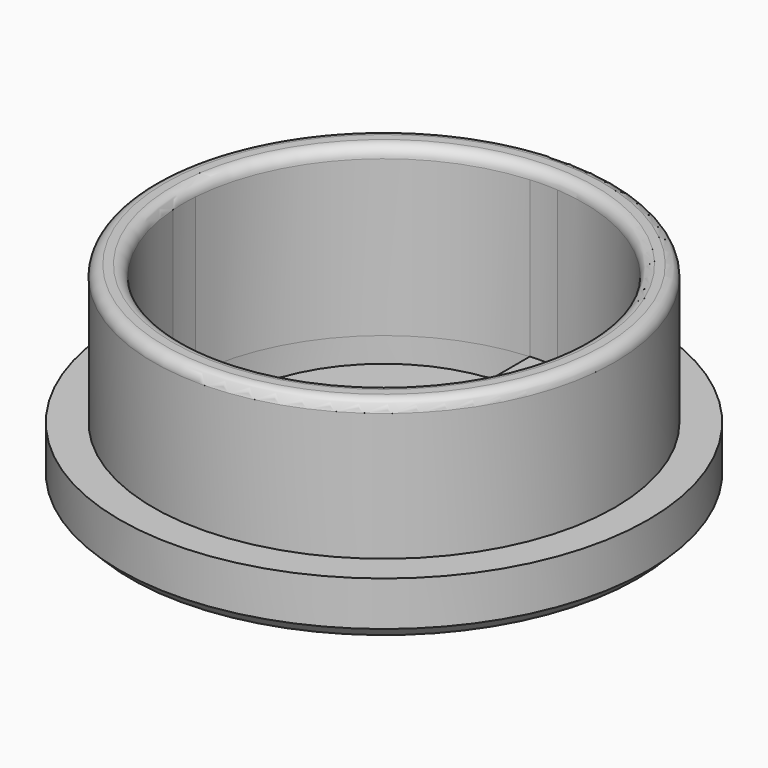
from build123d import *
from build123d import SkipClean  # not in build123d's __all__

# Parameters (mm, degrees)
F0_R     = 41.5
F0_R_2   = 36
F1_DEPTH = 35
F0_R_3   = 47.5
F2_DEPTH = 10
F3_DEPTH = 5
F4_R     = 2
F5_SIZE  = 2
F7_DEPTH = 40.1


with BuildPart() as f1:
    # F0 (on Top) → F1 (new body)
    with BuildSketch(Plane.XY):
        Circle(F0_R)
        Circle(F0_R_2, mode=Mode.SUBTRACT)
    extrude(amount=F1_DEPTH)

    # F0 (on Top) → F2 (join)
    with BuildSketch(Plane.XY):
        Circle(F0_R_3)
        Circle(F0_R, mode=Mode.SUBTRACT)
    extrude(amount=F2_DEPTH)

    # F0 (on Top) → F3 (join)
    with BuildSketch(Plane.XY):
        Circle(F0_R_2)
    extrude(amount=F3_DEPTH)

    # F4
    f4_edges = [f1.edges().sort_by_distance(p)[0] for p in [
        (-41.5, 0, 35),
        (-36, 0, 35),
    ]]
    fillet(f4_edges, radius=F4_R)

    # F5
    f5_edges = [f1.edges().sort_by_distance(p)[0] for p in [
        (-47.5, 0, 0),
    ]]
    chamfer(f5_edges, length=F5_SIZE)

    # F6 (on face) → F7 (cut)
    with BuildSketch(Plane.XY):
        with BuildLine():
            ThreePointArc((27.3098579389, -2.5), (19.3917294309, -19.3917294309), (2.5, -27.3098579389))
            Line((2.5, -27.3098579389), (2.5, -35.9130895357))
            ThreePointArc((2.5, -35.9130895357), (25.4558441227, -25.4558441227), (35.9130895357, -2.5))
            Line((35.9130895357, -2.5), (27.3098579389, -2.5))
        make_face()
        with BuildLine():
            Line((-2.5, -35.9130895357), (-2.5, -27.3098579389))
            ThreePointArc((-2.5, -27.3098579389), (-19.3917294309, -19.3917294309), (-27.3098579389, -2.5))
            Line((-27.3098579389, -2.5), (-35.9130895357, -2.5))
            ThreePointArc((-35.9130895357, -2.5), (-25.4558441227, -25.4558441227), (-2.5, -35.9130895357))
        make_face()
        with BuildLine():
            ThreePointArc((-27.3098579389, 2.5), (-19.3917294309, 19.3917294309), (-2.5, 27.3098579389))
            Line((-2.5, 27.3098579389), (-2.5, 35.9130895357))
            ThreePointArc((-2.5, 35.9130895357), (-25.4558441227, 25.4558441227), (-35.9130895357, 2.5))
            Line((-35.9130895357, 2.5), (-27.3098579389, 2.5))
        make_face()
        with BuildLine():
            Line((2.5, 35.9130895357), (2.5, 27.3098579389))
            ThreePointArc((2.5, 27.3098579389), (19.3917294309, 19.3917294309), (27.3098579389, 2.5))
            Line((27.3098579389, 2.5), (35.9130895357, 2.5))
            ThreePointArc((35.9130895357, 2.5), (25.4558441227, 25.4558441227), (2.5, 35.9130895357))
        make_face()
        with BuildLine():
            Line((2.5, 17.8404992818), (2.5, 8.7134999292))
            ThreePointArc((2.5, 8.7134999292), (6.4099563577, 6.4099563577), (8.7134999292, 2.5))
            Line((8.7134999292, 2.5), (17.8404992818, 2.5))
            ThreePointArc((17.8404992818, 2.5), (12.7383950053, 12.7383950053), (2.5, 17.8404992818))
        make_face()
        with BuildLine():
            ThreePointArc((8.7134999292, -2.5), (6.4099563577, -6.4099563577), (2.5, -8.7134999292))
            Line((2.5, -8.7134999292), (2.5, -17.8404992818))
            ThreePointArc((2.5, -17.8404992818), (12.7383950053, -12.7383950053), (17.8404992818, -2.5))
            Line((17.8404992818, -2.5), (8.7134999292, -2.5))
        make_face()
        with BuildLine():
            Line((-2.5, -17.8404992818), (-2.5, -8.7134999292))
            ThreePointArc((-2.5, -8.7134999292), (-6.4099563577, -6.4099563577), (-8.7134999292, -2.5))
            Line((-8.7134999292, -2.5), (-17.8404992818, -2.5))
            ThreePointArc((-17.8404992818, -2.5), (-12.7383950053, -12.7383950053), (-2.5, -17.8404992818))
        make_face()
        with BuildLine():
            ThreePointArc((-8.7134999292, 2.5), (-6.4099563577, 6.4099563577), (-2.5, 8.7134999292))
            Line((-2.5, 8.7134999292), (-2.5, 17.8404992818))
            ThreePointArc((-2.5, 17.8404992818), (-12.7383950053, 12.7383950053), (-17.8404992818, 2.5))
            Line((-17.8404992818, 2.5), (-8.7134999292, 2.5))
        make_face()
    with SkipClean():  # cleaning this boolean's faces spoils the solid; the shape is the same uncleaned
        extrude(amount=F7_DEPTH, mode=Mode.SUBTRACT)


solid = f1.part
